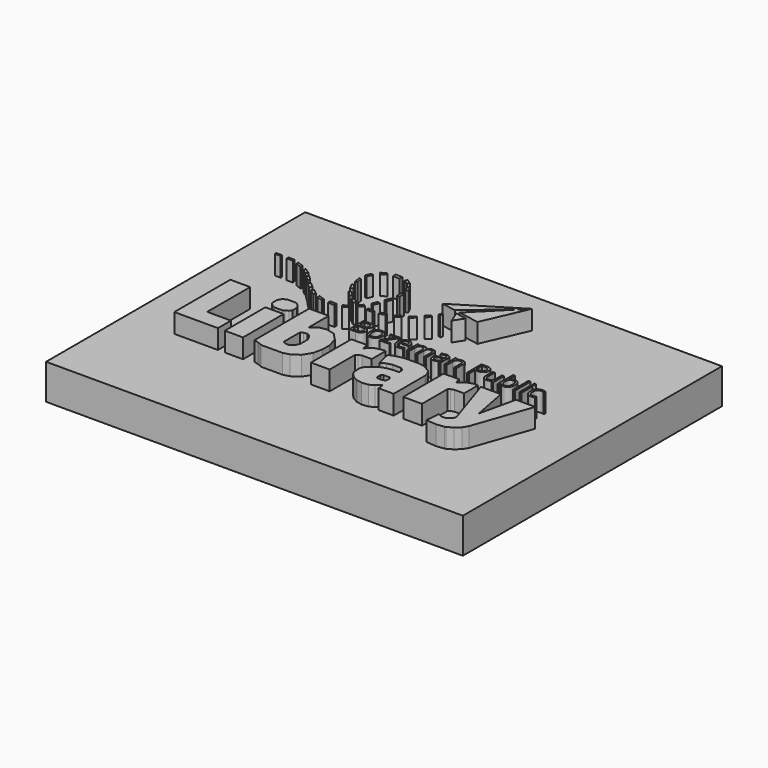
from build123d import *

# Parameters (mm, degrees)
F0_W         = 65
F0_H         = 50.5
F1_DEPTH     = 5.5
F2_W         = 2.8429944068
F2_H         = 7.9088687198
F2_W_2       = 0.8964985609
F2_H_2       = 0.256142579
F2_TEXT_SIZE = 3.9586616266
F3_DEPTH     = 3


# Not quite as in the source:
# - a feature names something its author has since deleted; it is built from what else it names
# - Text() gives the source's letters only with a copy of the font that has no kerning and outlines rounded to 1/6400 em; it was checked with that copy


with BuildPart() as f1:
    # F0 (on Top) → F1 (new body)
    with BuildSketch(Plane.XY):
        with Locations((-0.5076788366, -0.0209488949)):
            Rectangle(F0_W, F0_H)
    extrude(amount=F1_DEPTH)

    # F2 (on face) → F3 (join)
    with BuildSketch(Plane.XY.offset(5.5)):
        Polygon((-22.3070979118, 1.1384990066), (-25.4039317369, 1.1384990066), (-25.4039317369, -9.7765708342), (-18.6010506004, -9.7765708342), (-18.6010506004, -7.2381827049), (-22.3070979118, -7.2381827049), (-22.3070979118, 1.036963542), align=None)
        with Locations((-16.1073328927, -5.8221364743)):
            Rectangle(F2_W, F2_H)
        Polygon((-15.3996637091, 1.3987461571), (-16.629178077, 1.3987461571), (-17.1168437098, 1.2049939151), (-17.4329003533, 0.9051455418), (-17.6163800061, 0.492315914), (-17.6163800061, -0.4769364023), (-17.3291936517, -0.7820713799), (-16.9320697114, -1.0602826951), (-16.629178077, -1.1949010659), (-15.3996637091, -1.1949010659), (-15.1035031304, -1.0602826951), (-14.6906739101, -0.7820713799), (-14.44836054, -0.4769364023), (-14.44836054, 0.492315914), (-14.7445211187, 0.9051455418), (-15.0765795261, 1.2551533291), align=None)
        Polygon((-10.0961363658, 1.1909238528), (-13.1502393633, 1.1909238528), (-13.1502393633, -9.4529017806), (-12.4502237886, -9.6323927864), (-11.7207863654, -9.9565868755), (-8.4116728976, -9.9565868755), (-7.4065225199, -9.6862409264), (-6.2792572348, -8.9265612766), (-5.4859668016, -7.6759397052), (-5.1628830843, -6.1682136729), (-5.1628830843, -4.8040808178), (-5.6295599788, -3.2066097483), (-6.6765210171, -2.1030553485), (-8.034741506, -1.7527312739), (-8.9860446751, -1.9322223961), (-10.0961363658, -2.6803285234), align=None)
        Polygon((-10.0961363658, -7.6400414109), (-10.0961363658, -4.4271494262), (-9.7141868318, -4.2170494486), (-9.1810121051, -4.1164504669), (-8.7522138107, -4.3070272978), (-8.3999424901, -4.829751884), (-8.1831677965, -5.3066564724), (-8.1831677965, -6.7344547131), (-8.4058633393, -7.2355201808), (-8.7247055481, -7.6370246881), (-9.147586301, -7.8292431063), (-9.6704321293, -7.8292431063), align=None, mode=Mode.SUBTRACT)
        Polygon((-1.6997318016, -1.8945108168), (-4.086964298, -1.9304089947), (-4.086964298, -9.7921220586), (-1.1612583185, -9.7921220586), (-1.1612583185, -4.8202169128), (-0.8920215187, -4.622776527), (-0.4073954187, -4.4432855211), (1.1182794115, -4.4432855211), (1.1182794115, -1.7329689581), (0.4721111909, -1.7329689581), (-0.4612426274, -2.0022056997), (-0.9817670798, -2.3970860057), (-1.4125457965, -2.8637631331), align=None)
        Polygon((2.4004089646, -2.1828084718), (1.9539420027, -2.4178461172), (2.4662269279, -4.6377484687), (2.7137163561, -4.4493903406), (3.249950707, -4.211416468), (4.0334464595, -4.0306098381), (5.3687333129, -4.0306098381), (5.7114157826, -4.2843953706), (5.8827572502, -4.5763100497), (5.8827572502, -5.0649498589), (5.0450889394, -5.0649498589), (3.9472361095, -5.2109071985), (2.8874590062, -5.6360871531), (1.7769139959, -6.5562529489), (1.4887535945, -7.1539189667), (1.4887535945, -8.2986438647), (1.7769139959, -8.8933017105), (2.2854283452, -9.431774728), (3.1559604686, -9.8984520882), (4.0334464595, -10.0779430941), (5.0585670397, -9.9522992969), (5.7406332344, -9.5753679052), (6.4585977234, -8.9740725234), (6.5662926063, -9.3779275194), (6.5662926063, -9.9253756925), (8.9266011491, -9.9253756925), (8.9266011491, -3.8581702393), (8.7999887764, -3.2393429428), (8.4679350257, -2.6507023722), (7.8340135515, -2.2431819234), (7.1246265434, -1.8960350426), (6.2039326876, -1.7601947766), (4.2267041281, -1.7601947766), (3.4116632305, -1.8960350426), align=None)
        Polygon((5.8819521219, -6.8473231759), (6.0279094614, -7.1025500074), (6.0279094614, -7.7688773163), (5.5265780538, -7.9592559487), (4.860250745, -7.9592559487), (4.593720194, -7.7434931882), (4.593720194, -7.096204441), (4.8940941575, -6.8473231759), align=None, mode=Mode.SUBTRACT)
        Polygon((12.7383876847, -1.9399933786), (10.3511551883, -1.9758915564), (10.3511551883, -9.8376046204), (13.2768611679, -9.8376046204), (13.2768611679, -4.8656994746), (13.5460979677, -4.6682590887), (14.0307240676, -4.4887680829), (15.5563988978, -4.4887680829), (15.5563988978, -1.7784515199), (14.9102306773, -1.7784515199), (13.976876859, -2.0476882615), (13.4563524066, -2.4425685674), (13.0255736899, -2.9092456948), align=None)
        Polygon((19.1934686154, -1.853666734), (16.0703230649, -1.853666734), (18.761601299, -10.0645152852), (18.5374747962, -10.352675803), (18.2279702276, -10.7048712671), (17.7797209471, -10.9610138461), (17.0753281564, -10.9610138461), (16.8725494295, -10.843615979), (16.5648678091, -10.6356878012), (16.3816083223, -12.8500657156), (17.9291367531, -12.9781374708), (19.1934686154, -12.8500657156), (19.3370617926, -12.784678489), (20.1986189932, -12.3000526801), (20.9524817765, -11.617985554), (21.419160068, -10.8461743221), (24.5423056185, -1.853666734), (21.5448029339, -1.853666734), (20.2704146504, -7.4896891601), align=None)
        Polygon((5.0585670397, 11.2245902419), (8.0669308081, 18.0811528116), (-1.2424100275, 12.3452780702), (0.9590811096, 11.9425551966), (7.5464067049, 17.5606273115), (1.8206388922, 11.816910468), align=None)
        Polygon((3.3624790049, 11.0712455393), (1.64114777, 11.3861318678), (2.3950103205, 9.5553221181), align=None)
        with Locations((-24.9769315124, 10.0044352002)):
            Rectangle(F2_W_2, F2_H_2)
        Polygon((-22.6041954011, 10.1432520896), (-23.5475301743, 10.1583460346), (-23.5475301743, 9.8111983389), (-22.6041954011, 9.8111983389), align=None)
        Polygon((-20.8382736892, 9.5168780535), (-21.7514205724, 9.8262922838), (-21.7514205724, 9.5093315467), (-20.8382736892, 9.1169048101), align=None)
        Polygon((-19.1025380045, 8.5056237876), (-20.0307797641, 9.1018108651), (-20.0307797641, 8.6942911148), (-19.4421391934, 8.2188500091), align=None)
        Polygon((-18.5163095593, 7.9258251935), (-18.8145693392, 7.6846778393), (-18.0256684422, 6.9270004521), (-17.7801772952, 7.1643083356), align=None)
        Polygon((-17.1917290277, 6.5984499191), (-17.4764785916, 6.3231922686), (-16.6650756843, 5.5319965431), (-16.3595881313, 5.891666282), align=None)
        Polygon((-14.9390520767, 4.7791066237), (-15.7249905169, 5.4093725048), (-16.0213296472, 5.1229116173), (-15.1411611587, 4.495552741), align=None)
        Polygon((-13.288137503, 4.2544058524), (-14.2273409292, 4.5590125956), (-14.2273409292, 4.1782543994), (-13.288137503, 3.8990315516), align=None)
        Polygon((-12.3489340767, 4.2913770303), (-12.3489340767, 3.8355719298), (-11.3208862022, 3.8355719298), (-11.3208862022, 4.2670979165), align=None)
        Polygon((-10.2789774537, 3.9952164516), (-9.6161747351, 4.5590125956), (-9.8259388957, 4.7760102089), (-10.5985393748, 4.4700363651), align=None)
        Polygon((-8.2056463198, 5.8898971103), (-8.5792634636, 6.1572529376), (-9.2227411103, 5.535225136), (-8.8574746624, 5.259796977), align=None)
        Polygon((-6.5420386381, 5.690576043), (-7.5561637059, 5.699550733), (-7.5561637059, 5.286721047), (-6.5420386381, 5.286721047), align=None)
        Polygon((-4.8368731514, 5.699550733), (-4.9355928786, 6.0585327446), (-5.7433033362, 5.7892962359), (-5.7433033362, 5.4093725048), align=None)
        Polygon((-7.2843873144, 7.6846778393), (-7.6997568831, 7.7816480771), (-8.0766882747, 6.9829123095), (-7.6995465768, 6.8049353729), align=None)
        Polygon((-10.3846024722, 6.6509479422), (-10.7780303806, 6.408540532), (-9.9690763699, 5.7493268138), (-9.7010834143, 6.0585327446), align=None)
        Polygon((-6.618284005, 9.410284691), (-7.0401695557, 9.5587624237), (-7.3722233064, 8.6942911148), (-6.9948895834, 8.5324151441), align=None)
        Polygon((-6.5119024366, 11.4303370938), (-6.9194226526, 11.4454310387), (-6.9194226526, 10.4794567451), (-6.5119024366, 10.4794567451), align=None)
        Polygon((-11.9224452648, 7.9258251935), (-12.1719082817, 7.6846778393), (-11.4602692808, 6.8994841828), (-11.1863130006, 7.1643083356), align=None)
        Polygon((-12.7986435826, 9.5587624237), (-13.0926016718, 9.3776425347), (-12.6398010179, 8.5173211992), (-12.2660066072, 8.6942911148), align=None)
        Polygon((-2.9581362189, 6.408540532), (-3.1913660932, 6.7363064736), (-3.9952937031, 6.2409730067), (-3.709663437, 5.9454931407), align=None)
        Polygon((-1.3801644091, 7.5362538919), (-1.6518445918, 7.7816480771), (-2.4065119214, 7.1643083356), (-2.1197383758, 6.8796933629), align=None)
        Polygon((0.5702277921, 10.1583460346), (0.28556303, 10.3304665536), (0.145951868, 9.8262922838), (0.4546108183, 9.7408213717), align=None)
        Polygon((-0.0539844706, 8.8020019862), (-0.4124937695, 9.1018108651), (-1.0326483737, 8.5023286499), (-0.7096502457, 8.1681923383), align=None)
        Polygon((-13.0926016718, 11.2581728026), (-13.3900856599, 11.2581728026), (-13.3940121159, 11.2232547253), (-13.2377696058, 10.2658412942), (-12.9077918828, 10.3316614404), align=None)
        Polygon((-12.6073869568, 12.9900914805), (-12.9542490467, 13.1093515083), (-13.3132310584, 12.3016415164), (-12.9793218422, 12.1532375058), align=None)
        Polygon((-11.6140982136, 14.4548984244), (-12.3410373926, 13.9612974599), (-12.0538510382, 13.6471875012), (-11.2999882549, 14.1946356744), align=None)
        Polygon((-9.4871278852, 14.7779826075), (-10.5371512473, 14.7869568318), (-10.5371512473, 14.248482883), (-9.4871278852, 14.248482883), align=None)
        Polygon((-8.4438389167, 14.5385218784), (-8.7355123833, 14.2737729475), (-7.9951109365, 13.7936342508), (-7.7393362299, 14.0628702939), align=None)
        Polygon((-7.1053862703, 13.2689133143), (-7.4085537344, 13.1093515083), (-6.9603039883, 12.2680533677), (-6.6981075359, 12.4950836352), align=None)
        with Locations((-6.3424801435, 0)):
            Text('Bozeman Public', F2_TEXT_SIZE, font='Open Sans', text_align=(TextAlign.LEFT, TextAlign.BOTTOM))
    extrude(amount=F3_DEPTH)


solid = f1.part
